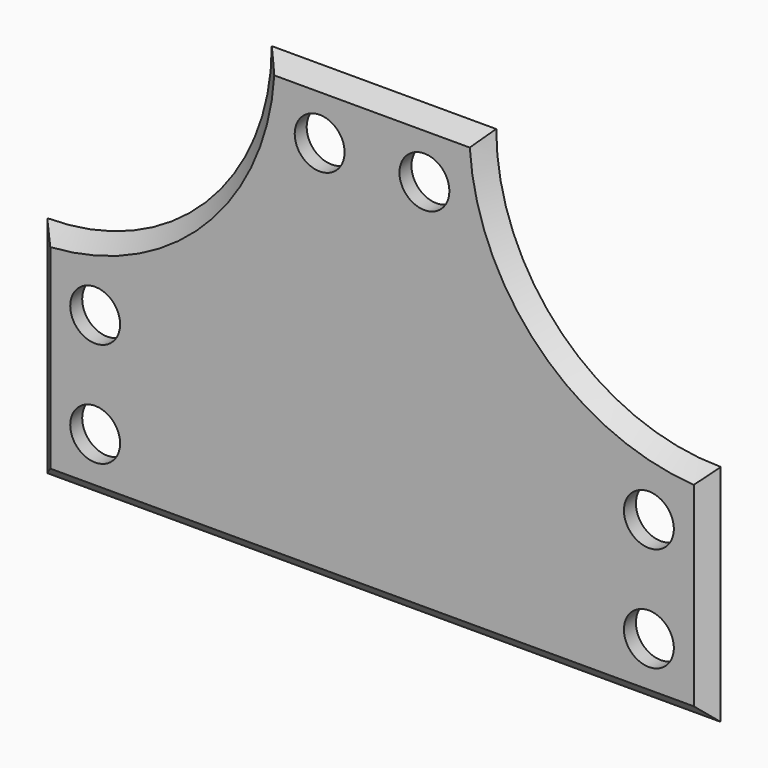
from build123d import *

# Parameters (mm, degrees)
F1_DEPTH = 3
F3_D     = 10
F3_DEPTH = 9
F3_TIP   = 3.0043030951
F4_SIZE  = 2.99999


# Not quite as in the source:
# - a fillet or chamfer is up to 0.001 mm smaller than in the source, because OpenCascade refuses the exact size


with BuildPart() as f1:
    # F0 (on Front) → F1 (new body)
    with BuildSketch(Plane.XZ):
        with BuildLine():
            Line((0, 45), (0, 0))
            Line((0, 0), (135, 0))
            Line((135, 0), (135, 45))
            ThreePointArc((135, 45), (103.1801948466, 58.1801948466), (90, 90))
            Line((90, 90), (45, 90))
            ThreePointArc((45, 90), (31.8198051534, 58.1801948466), (0, 45))
        make_face()
    extrude(amount=F1_DEPTH)

    # F3
    with Locations(Plane.XZ.offset(3)):
        with Locations((57, 78), (78, 78), (123, 33), (123, 12), (12, 12), (12, 33)):
            Hole(F3_D / 2, depth=F3_DEPTH)
            with Locations((0, 0, -(F3_DEPTH + F3_TIP / 2))):  # 118° drill point
                Cone(0, F3_D / 2, F3_TIP, mode=Mode.SUBTRACT)

    # F4 (size 3 in the source; OpenCascade refuses exactly that, so slightly less here)
    f4_edges = [f1.edges().sort_by_distance(p)[0] for p in [
        (31.819805, -3, 58.180195),
        (67.5, -3, 90),
        (103.180195, -3, 58.180195),
        (135, -3, 22.5),
        (0, -3, 22.5),
        (67.5, -3, 0),
    ]]
    chamfer(f4_edges, length=F4_SIZE)


solid = f1.part
